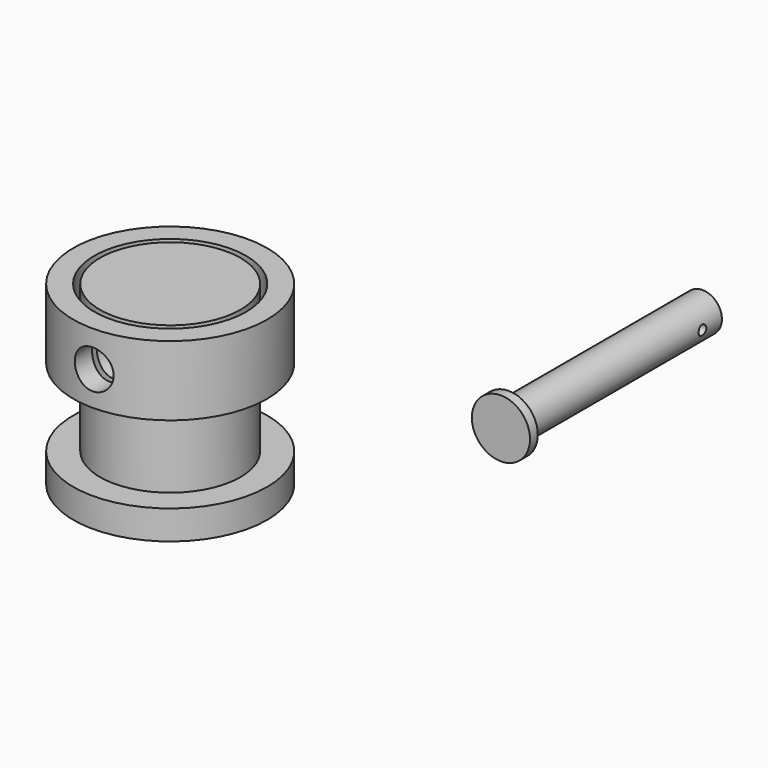
from build123d import *

# Parameters (mm, degrees)
F0_R          = 10
F0_R_2        = 7.83
F1_DEPTH      = 7
F1_DEPTH_BACK = 0.2
F3_R          = 7.25
F4_DEPTH      = 7.2
F4_DEPTH_BACK = 8
F5_START      = 8
F3_R_2        = 10
F3_R_3        = 7.83
F5_DEPTH      = 3
F2_R          = 2
F10_DEPTH     = 93.8892550597
F7_R          = 2
F11_DEPTH     = 25
F7_R_2        = 3
F12_DEPTH     = 1
F13_R         = 0.5
F14_DEPTH     = 25


# Not quite as in the source:
# - a feature of the source that left no trace in its solid (it failed there, or was rolled back) is left out


with BuildPart() as f1:
    # F0 (on Top) → F1 (new body, two sides)
    with BuildSketch(Plane.XY) as f1_sk:
        with Locations((-31.695947051, 83.8882550597)):
            Circle(F0_R)
        with Locations((-31.695947051, 83.8882550597)):
            Circle(F0_R_2, mode=Mode.SUBTRACT)
    extrude(amount=F1_DEPTH)
    extrude(f1_sk.sketch, amount=-F1_DEPTH_BACK)


with BuildPart() as f4:
    # F3 (on face) → F4 (new body, two sides)
    with BuildSketch(Plane(origin=(0, 0, -0.2), x_dir=(1, 0, 0), z_dir=(0, 0, -1))) as f4_sk:
        with Locations((-31.695947051, -83.8882550597)):
            Circle(F3_R)
    extrude(amount=-F4_DEPTH)
    extrude(f4_sk.sketch, amount=F4_DEPTH_BACK)

    # F3 (on face) → F5 (join)
    with BuildSketch(Plane(origin=(0, 0, -0.2), x_dir=(1, 0, 0), z_dir=(0, 0, -1)).offset(F5_START)):
        with Locations((-31.695947051, -83.8882550597)):
            Circle(F3_R_2)
        with Locations((-31.695947051, -83.8882550597)):
            Circle(F3_R_3, mode=Mode.SUBTRACT)
        with Locations((-31.695947051, -83.8882550597)):
            Circle(F3_R_3)
        with Locations((-31.695947051, -83.8882550597)):
            Circle(F3_R, mode=Mode.SUBTRACT)
        with Locations((-31.695947051, -83.8882550597)):
            Circle(F3_R)
    extrude(amount=F5_DEPTH)


with BuildPart() as f10_tool:
    # F2 (on Front) → F10 (new body, through all)
    with BuildSketch(Plane.XZ):
        with Locations((-31.695947051, 3.3)):
            Circle(F2_R)
    extrude(amount=-F10_DEPTH)


with BuildPart() as f1_1:
    add(f1.part)

    # F10: cut by f10_tool
    add(f10_tool.part, mode=Mode.SUBTRACT)


with BuildPart() as f4_1:
    add(f4.part)

    # F10: cut by f10_tool
    add(f10_tool.part, mode=Mode.SUBTRACT)


with BuildPart() as f11:
    # F7 (on offset) → F11 (new body)
    with BuildSketch(Plane.XZ.offset(-70)):
        with Locations((14.3349738792, 14.8918386549)):
            Circle(F7_R)
    extrude(amount=-F11_DEPTH)

    # F7 (on offset) → F12 (join)
    with BuildSketch(Plane.XZ.offset(-70)):
        with Locations((14.3349738792, 14.8918386549)):
            Circle(F7_R_2)
        with Locations((14.3349738792, 14.8918386549)):
            Circle(F7_R, mode=Mode.SUBTRACT)
        with Locations((14.3349738792, 14.8918386549)):
            Circle(F7_R)
    extrude(amount=F12_DEPTH)

    # F13 (on Right) → F14 (cut)
    with BuildSketch(Plane.YZ):
        with Locations((92.5, 14.8918386549)):
            Circle(F13_R)
    extrude(amount=F14_DEPTH, mode=Mode.SUBTRACT)


solid = Compound([f1_1.part, f4_1.part, f11.part])
